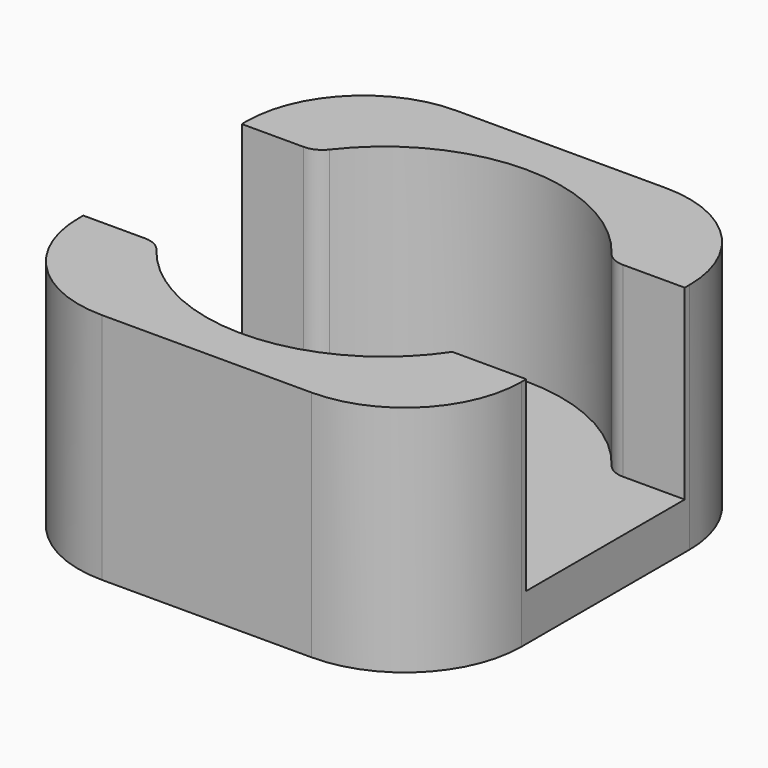
from build123d import *

# Parameters (mm, degrees)
F0_W     = 19
F0_H     = 19
F1_DEPTH = 2
F3_DEPTH = 8
F4_R     = 5
F5_R     = 1


with BuildPart() as f1:
    # F0 (on Top) → F1 (new body)
    with BuildSketch(Plane.XY):
        Rectangle(F0_W, F0_H)
    extrude(amount=F1_DEPTH)

    # F2 (on face) → F3 (join)
    with BuildSketch(Plane.XY.offset(2)):
        with BuildLine():
            Line((9.5, -4.25), (6.3307286311, -4.25))
            ThreePointArc((6.3307286311, -4.25), (0, -7.625), (-6.3307286311, -4.25))
            Line((-6.3307286311, -4.25), (-9.5, -4.25))
            Line((-9.5, -4.25), (-9.5, -9.5))
            Line((-9.5, -9.5), (9.5, -9.5))
            Line((9.5, -9.5), (9.5, -4.25))
        make_face()
        with BuildLine():
            ThreePointArc((-6.3307286311, 4.25), (0, 7.625), (6.3307286311, 4.25))
            Line((6.3307286311, 4.25), (9.5, 4.25))
            Line((9.5, 4.25), (9.5, 9.5))
            Line((9.5, 9.5), (-9.5, 9.5))
            Line((-9.5, 9.5), (-9.5, 4.25))
            Line((-9.5, 4.25), (-6.3307286311, 4.25))
        make_face()
    extrude(amount=F3_DEPTH)

    # F4
    f4_edges = [f1.edges().sort_by_distance(p)[0] for p in [
        (-9.5, -9.5, 5),
        (9.5, -9.5, 5),
        (9.5, 9.5, 5),
        (-9.5, 9.5, 5),
    ]]
    fillet(f4_edges, radius=F4_R)

    # F5
    f5_edges = [f1.edges().sort_by_distance(p)[0] for p in [
        (6.330729, 4.25, 6),
        (-6.330729, 4.25, 6),
        (-6.330729, -4.25, 6),
    ]]
    fillet(f5_edges, radius=F5_R)


solid = f1.part
